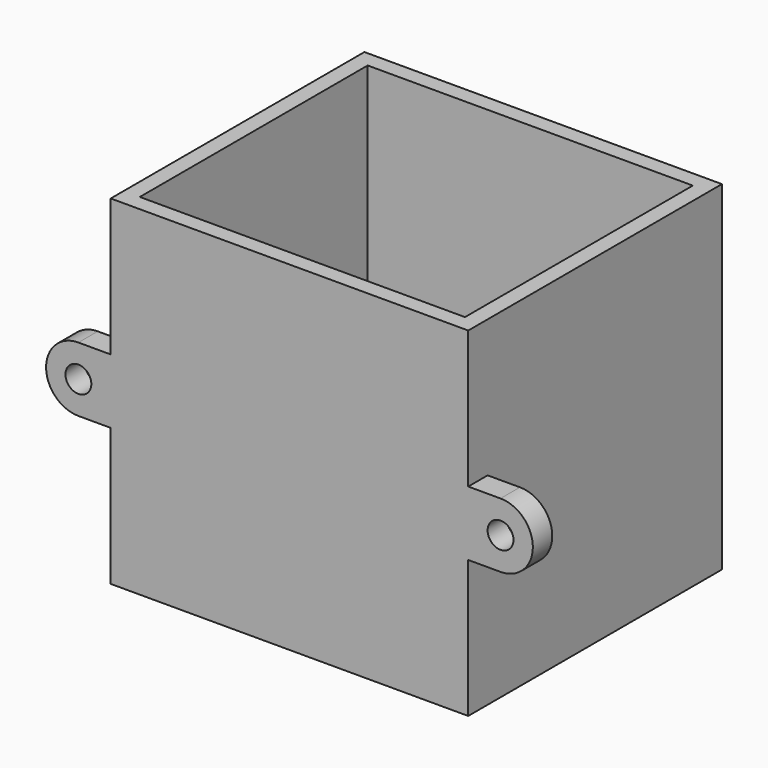
from build123d import *

# Parameters (mm, degrees)
F0_W     = 63.896875
F0_H     = 55.959375
F1_DEPTH = 66.675
F2_W     = 63.896875
F2_H     = 55.959375
F3_DEPTH = 3.175
F4_R     = 2.54
F5_DEPTH = 4.7625


# Not quite as in the source:
# - a pattern or mirror of a feature is missing from the dataset's text; its kind, count and spacing are read off the source's solid


with BuildPart() as f1:
    # F0 (on Top) → F1 (new body)
    with BuildSketch(Plane.XY):
        Polygon((35.1234375, -31.1546875), (35.1234375, 31.1546875), (-35.1234375, 31.1546875), (-35.1234375, -31.1546875), align=None)
        Rectangle(F0_W, F0_H, mode=Mode.SUBTRACT)
    extrude(amount=F1_DEPTH)

    # F2 (on Top) → F3 (join)
    with BuildSketch(Plane.XY):
        Rectangle(F2_W, F2_H)
        with BuildLine():
            ThreePointArc((-27.1859375, 6.1708083338), (0, 26.3921875), (27.1859375, 6.1708083338))
            Line((27.1859375, 6.1708083338), (0, -9.525))
            Line((0, -9.525), (-27.1859375, 6.1708083338))
        make_face(mode=Mode.SUBTRACT)
    extrude(amount=F3_DEPTH)

    # F4 (on face) → F5 (join)
    with BuildSketch(Plane.XZ.offset(31.1546875)):
        with BuildLine():
            Line((-35.1234375, 26.9875), (-35.1234375, 39.6875))
            Line((-35.1234375, 39.6875), (-41.4734375, 39.6875))
            ThreePointArc((-41.4734375, 39.6875), (-47.8234375, 33.3375), (-41.4734375, 26.9875))
            Line((-41.4734375, 26.9875), (-35.1234375, 26.9875))
        make_face()
        with Locations((-41.4734375, 33.3375)):
            Circle(F4_R, mode=Mode.SUBTRACT)
    f5 = extrude(amount=-F5_DEPTH)

    # F5_copies: F5 across plane
    add(f5.mirror(Plane(origin=(0, 0, 0), x_dir=(0, 0, 1), z_dir=(1, 0, 0))))


solid = f1.part
